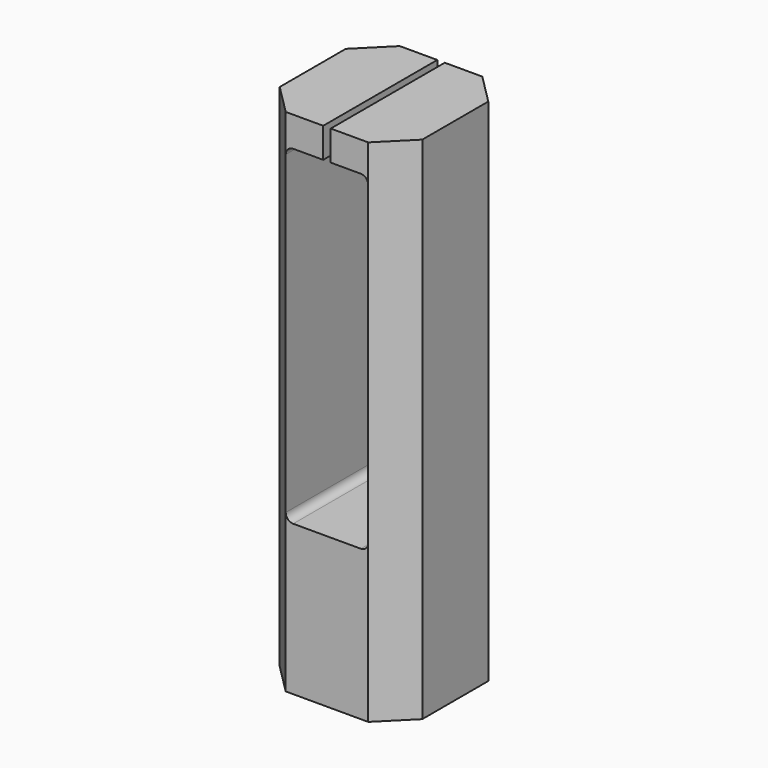
from build123d import *

# Parameters (mm, degrees)
F0_W      = 9.5
F0_H      = 10
F1_DEPTH  = 9.5
F3_DEPTH  = 9.5
F8_SIZE   = 1.99999
F10_D     = 2.8
F10_DEPTH = 5
F10_TIP   = 0.8412048666
F11_R     = 0.5


# Not quite as in the source:
# - a fillet or chamfer is up to 0.001 mm smaller than in the source, because OpenCascade refuses the exact size


with BuildPart() as f1:
    # F0 (on Front) → F1 (new body)
    with BuildSketch(Plane.XZ):
        with Locations((4.75, 5)):
            Rectangle(F0_W, F0_H)
    extrude(amount=F1_DEPTH)

    # F2 (on Front) → F3 (join)
    with BuildSketch(Plane.XZ):
        Polygon((7.5, 10), (9.5, 10), (9.5, 34), (5, 34), (5, 32), (7.5, 32), align=None)
    extrude(amount=F3_DEPTH)


with BuildPart() as f5_1:
    # F5: instance of F1
    add(f1.part.mirror(Plane(origin=(4.75, -4.75, 5), x_dir=(0, -1, 0), z_dir=(-1, 0, 0))))


with BuildPart() as f1_1:
    add(f1.part)

    # F6: union 

    # F7: union F5_1
    add(f5_1.part)

    # F8 (size 2 in the source; OpenCascade refuses exactly that, so slightly less here)
    f8_edges = [f1_1.edges().sort_by_distance(p)[0] for p in [
        (9.5, -9.5, 17),
        (9.5, 0, 17),
        (0, -9.5, 17),
        (0, 0, 17),
    ]]
    chamfer(f8_edges, length=F8_SIZE)

    # F10
    with Locations(Plane(origin=(0, 0, 0), x_dir=(1, 0, 0), z_dir=(0, 0, -1))):
        with Locations((4.75, 4.75)):
            Hole(F10_D / 2, depth=F10_DEPTH)
            with Locations((0, 0, -(F10_DEPTH + F10_TIP / 2))):  # 118° drill point
                Cone(0, F10_D / 2, F10_TIP, mode=Mode.SUBTRACT)

    # F11
    f11_edges = [f1_1.edges().sort_by_distance(p)[0] for p in [
        (2, -4.75, 10),
        (7.5, -4.75, 10),
        (2, -4.75, 32),
        (7.5, -4.75, 32),
    ]]
    fillet(f11_edges, radius=F11_R)


solid = f1_1.part
